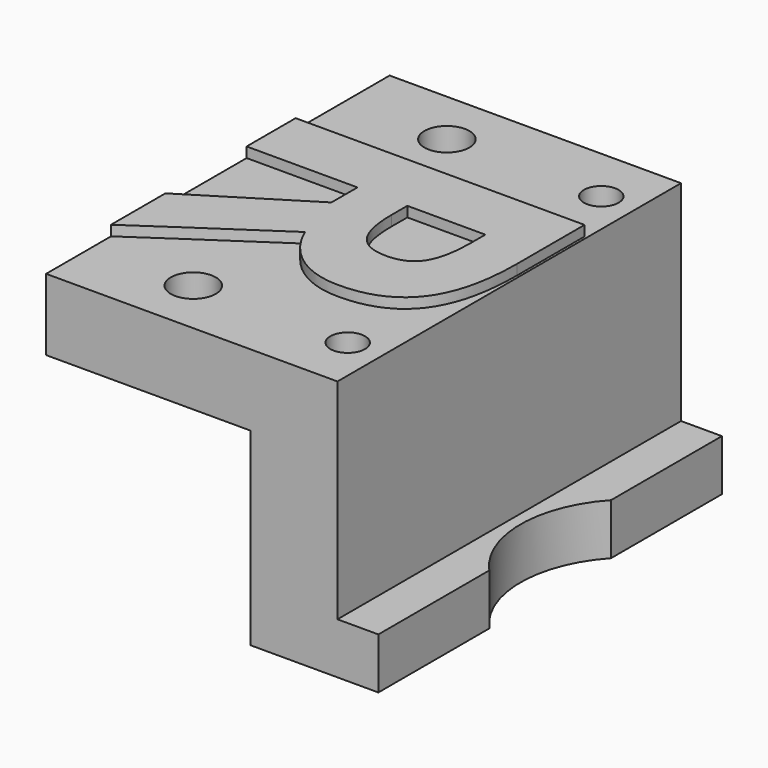
from build123d import *

# Parameters (mm, degrees)
F1_DEPTH     = 42
F2_R         = 1.7
F2_R_2       = 11
F3_DEPTH     = 25.481
F4_W         = 42
F4_H         = 7
F5_DEPTH     = 20
F6_R         = 2.2
F7_DEPTH     = 25
F8_TEXT_SIZE = 39.5833333333
F9_DEPTH     = 1


# Not quite as in the source:
# - Text() gives the source's letters only with a copy of the font that has no kerning and outlines rounded to 1/6400 em; it was checked with that copy


with BuildPart() as f1:
    # F0 (on Front) → F1 (new body)
    with BuildSketch(Plane.XZ):
        Polygon((8.5, 5), (8.5, 25.48), (0, 25.48), (0, 0), (12.5, 0), (12.5, 5), align=None)
    extrude(amount=-F1_DEPTH)

    # F2 (on face) → F3 (cut, through all)
    with BuildSketch(Plane(origin=(0, 0, 0), x_dir=(1, 0, 0), z_dir=(0, 0, -1))):
        with Locations((5.1, -5.5)):
            Circle(F2_R)
        with Locations((5.1, -36.5)):
            Circle(F2_R)
        with Locations((20.6, -21)):
            Circle(F2_R_2)
    extrude(amount=-F3_DEPTH, mode=Mode.SUBTRACT)

    # F4 (on face) → F5 (join)
    with BuildSketch(Plane(origin=(0, 0, 0), x_dir=(0, -1, 0), z_dir=(-1, 0, 0))):
        with Locations((-21, 21.98)):
            Rectangle(F4_W, F4_H)
    extrude(amount=F5_DEPTH)

    # F6 (on face) → F7 (cut)
    with BuildSketch(Plane.XY.offset(25.48)):
        with Locations((-10, 36.5)):
            Circle(F6_R)
        with Locations((-10, 5.5)):
            Circle(F6_R)
    extrude(amount=-F7_DEPTH, mode=Mode.SUBTRACT)

    # F8 (on face) → F9 (join)
    with BuildSketch(Plane.XY.offset(25.48)):
        with Locations(Location((-20, 34.0655924479), (0, 0, -90))):
            Text('R', F8_TEXT_SIZE, font='Open Sans', font_style=FontStyle.BOLD, text_align=(TextAlign.LEFT, TextAlign.BOTTOM))
    extrude(amount=F9_DEPTH)


solid = f1.part
